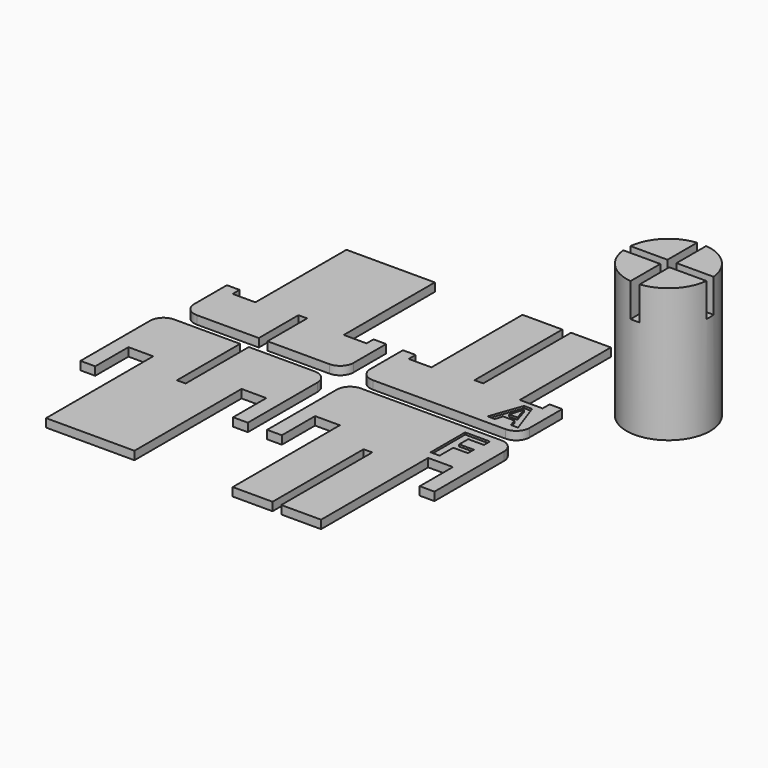
from build123d import *

# Parameters (mm, degrees)
F1_DEPTH     = 3.175
F2_TEXT_SIZE = 22.9708071048
F3_DEPTH     = 0.762
F5_DEPTH     = 3.175
F6_TEXT_SIZE = 16.7060410604
F7_DEPTH     = 0.762
F8_R         = 5.08
F8_2_R       = 5.08
F8_3_R       = 5.08
F8_4_R       = 5.08
F9_R         = 15.875
F10_DEPTH    = 50.8
F11_W        = 3.429
F11_H        = 14.1605
F11_H_2      = 3.429
F11_W_2      = 14.1605
F12_DEPTH    = 12.7


# Not quite as in the source:
# - Text() gives the source's letters only with a copy of the font that has no kerning and outlines rounded to 1/6400 em; it was checked with that copy


with BuildPart() as f1:
    # F0 (on Top) → F1 (new body)
    with BuildSketch(Plane.XY):
        Polygon((-37.0630887776, -29.972), (-37.0630887776, 0), (-67.1620887776, 0), (-67.1620887776, -38.1), (-61.5740887776, -38.1), (-61.5740887776, -22.352), (-52.1760887776, -22.352), (-52.1760887776, -73.152), (-35.4120887776, -73.152), (-18.6480887776, -73.152), (-18.6480887776, -22.352), (-9.2500887776, -22.352), (-9.2500887776, -38.1), (-3.6620887776, -38.1), (-3.6620887776, 0), (-33.7610887776, 0), (-33.7610887776, -29.972), (-35.4120887776, -29.972), align=None)
    extrude(amount=F1_DEPTH)

    # F8#3
    f8_3_edges = [f1.edges().sort_by_distance(p)[0] for p in [
        (-3.662089, 0, 1.5875),
        (-67.162089, 0, 1.5875),
    ]]
    fillet(f8_3_edges, radius=F8_3_R)


with BuildPart() as f1b:
    # F0 (on Top) → F1, piece 2 (new body)
    with BuildSketch(Plane.XY):
        Polygon((35.4120887776, 0), (3.6620887776, 0), (3.6620887776, -38.1), (9.2500887776, -38.1), (9.2500887776, -22.352), (18.6480887776, -22.352), (18.6480887776, -73.152), (33.7610887776, -73.152), (33.7610887776, -29.972), (37.0630887776, -29.972), (37.0630887776, -73.152), (52.1760887776, -73.152), (52.1760887776, -22.352), (61.5740887776, -22.352), (61.5740887776, -38.1), (67.1620887776, -38.1), (67.1620887776, 0), align=None)
    extrude(amount=F1_DEPTH)

    # F2 (on face) → F3 (cut)
    with BuildSketch(Plane.XY.offset(3.175)):
        with Locations((48.435587436, -19.1164836287)):
            Text('F', F2_TEXT_SIZE, font='Open Sans', font_style=FontStyle.BOLD, text_align=(TextAlign.LEFT, TextAlign.BOTTOM))
    extrude(amount=-F3_DEPTH, mode=Mode.SUBTRACT)

    # F8#2
    f8_2_edges = [f1b.edges().sort_by_distance(p)[0] for p in [
        (67.162089, 0, 1.5875),
        (3.662089, 0, 1.5875),
    ]]
    fillet(f8_2_edges, radius=F8_2_R)


with BuildPart() as f5:
    # F4 (on Top) → F5 (new body)
    with BuildSketch(Plane.XY):
        Polygon((-31.75, 6.35), (-3.175, 6.35), (-3.175, 26.924), (-8.001, 26.924), (-8.001, 23.622), (-16.637, 23.622), (-16.637, 66.802), (-33.401, 66.802), (-50.165, 66.802), (-50.165, 23.622), (-58.801, 23.622), (-58.801, 26.924), (-63.627, 26.924), (-63.627, 6.35), (-35.052, 6.35), (-35.052, 25.146), (-33.401, 25.146), (-31.75, 25.146), align=None)
    extrude(amount=F5_DEPTH)

    # F8#4
    f8_4_edges = [f5.edges().sort_by_distance(p)[0] for p in [
        (-63.627, 6.35, 1.5875),
        (-3.175, 6.35, 1.5875),
    ]]
    fillet(f8_4_edges, radius=F8_4_R)


with BuildPart() as f5b:
    # F4 (on Top) → F5, piece 2 (new body)
    with BuildSketch(Plane.XY):
        Polygon((3.175, 26.924), (3.175, 6.35), (63.627, 6.35), (63.627, 26.924), (58.801, 26.924), (58.801, 23.622), (50.165, 23.622), (50.165, 66.802), (35.052, 66.802), (35.052, 25.146), (33.401, 25.146), (31.75, 25.146), (31.75, 66.802), (16.637, 66.802), (16.637, 23.622), (8.001, 23.622), (8.001, 26.924), align=None)
    extrude(amount=F5_DEPTH)

    # F6 (on face) → F7 (cut)
    with BuildSketch(Plane.XY.offset(3.175)):
        with Locations((49.2947511375, 9.4508454204)):
            Text('A', F6_TEXT_SIZE, font='Open Sans', font_style=FontStyle.BOLD, text_align=(TextAlign.LEFT, TextAlign.BOTTOM))
    extrude(amount=-F7_DEPTH, mode=Mode.SUBTRACT)

    # F8
    f8_edges = [f5b.edges().sort_by_distance(p)[0] for p in [
        (3.175, 6.35, 1.5875),
        (63.627, 6.35, 1.5875),
    ]]
    fillet(f8_edges, radius=F8_R)


with BuildPart() as f10:
    # F9 (on Top) → F10 (new body)
    with BuildSketch(Plane.XY):
        with Locations((86.9954526424, 48.0735041201)):
            Circle(F9_R)
    extrude(amount=F10_DEPTH)

    # F11 (on face) → F12 (cut)
    with BuildSketch(Plane.XY.offset(50.8)):
        with Locations((86.9954526424, 56.8682541201)):
            Rectangle(F11_W, F11_H)
        with Locations((86.9954526424, 48.0735041201)):
            Rectangle(F11_W, F11_H_2)
        with Locations((78.2007026424, 48.0735041201)):
            Rectangle(F11_W_2, F11_H_2)
        with Locations((95.7902026424, 48.0735041201)):
            Rectangle(F11_W_2, F11_H_2)
        with Locations((86.9954526424, 39.2787541201)):
            Rectangle(F11_W, F11_H)
    extrude(amount=-F12_DEPTH, mode=Mode.SUBTRACT)


solid = Compound([f1.part, f1b.part, f5.part, f5b.part, f10.part])
